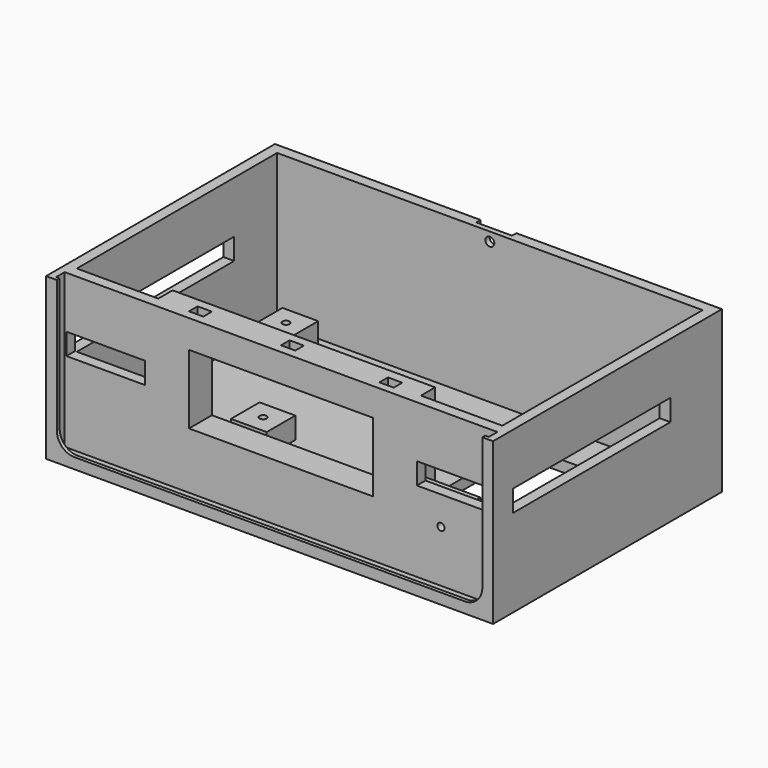
from build123d import *

# Parameters (mm, degrees)
F0_W      = 125
F0_H      = 80
F1_DEPTH  = 45
F3_DEPTH  = 4
F4_W      = 121
F4_H      = 46.7722373752
F5_DEPTH  = 3
F6_W      = 51.45
F6_H      = 19.35
F6_W_2    = 22
F6_H_2    = 6
F7_DEPTH  = 50
F9_DEPTH  = 42
F10_W     = 10
F10_H     = 10
F10_R     = 1
F11_DEPTH = 6
F12_W     = 55
F12_H     = 6
F13_DEPTH = 10
F14_W     = 55
F14_H     = 6
F15_DEPTH = 10
F16_W     = 27.3198820651
F16_H     = 40
F17_DEPTH = 25
F19_W     = 2
F19_H     = 1.5
F20_DEPTH = 5
F21_W     = 27.3198820651
F21_H     = 6
F22_DEPTH = 1.5
F24_R     = 1.5
F25_DEPTH = 10
F26_W     = 4
F26_H     = 3
F27_DEPTH = 5
F28_W     = 10
F28_H     = 10
F29_DEPTH = 1.5
F30_R     = 1.25
F31_DEPTH = 10
F32_W     = 15
F32_H     = 21
F33_DEPTH = 2
F34_R     = 1.4
F34_R_2   = 1.75
F35_DEPTH = 3
F36_R     = 1
F37_DEPTH = 25


# Not quite as in the source:
# - a feature names something its author has since deleted; it is built from what else it names


with BuildPart() as f1:
    # F0 (on Top) → F1 (new body)
    with BuildSketch(Plane.XY):
        Rectangle(F0_W, F0_H)
    extrude(amount=F1_DEPTH)

    # F2 (on face) → F3 (cut)
    with BuildSketch(Plane.XZ.offset(40)):
        with BuildLine():
            Line((-59.5, 47), (-59.5, 7.948817455))
            ThreePointArc((-59.5, 7.948817455), (-58.0505249263, 4.4494750737), (-54.551182545, 3))
            Line((-54.551182545, 3), (0, 3))
            Line((0, 3), (54.551182545, 3))
            ThreePointArc((54.551182545, 3), (58.0505249263, 4.4494750737), (59.5, 7.948817455))
            Line((59.5, 7.948817455), (59.5, 47))
            Line((59.5, 47), (0, 47))
            Line((0, 47), (-59.5, 47))
        make_face()
    extrude(amount=-F3_DEPTH, mode=Mode.SUBTRACT)

    # F4 (on face) → F5 (cut)
    with BuildSketch(Plane.XZ.offset(36)):
        with Locations((0, 25.3861186876)):
            Rectangle(F4_W, F4_H)
    extrude(amount=F5_DEPTH, mode=Mode.SUBTRACT)

    # F6 (on face) → F7 (cut)
    with BuildSketch(Plane.XZ.offset(36)):
        with Locations((0, 27.5)):
            Rectangle(F6_W, F6_H)
        with Locations((-49, 27.5)):
            Rectangle(F6_W_2, F6_H_2)
        with Locations((49, 27.5)):
            Rectangle(F6_W_2, F6_H_2)
    extrude(amount=-F7_DEPTH, mode=Mode.SUBTRACT)

    # F8 (on face) → F9 (cut)
    with BuildSketch(Plane.XY.offset(45)):
        Polygon((-36.725, -28), (0, -28), (0, 37), (-59.5, 37), (-59.5, -33), (-36.725, -33), align=None)
        Polygon((0, 37), (0, -28), (36.725, -28), (36.725, -33), (59.5, -33), (59.5, 37), align=None)
    extrude(amount=-F9_DEPTH, mode=Mode.SUBTRACT)

    # F10 (on face) → F11 (join)
    with BuildSketch(Plane.XY.offset(3)):
        with Locations((-51, 29.5)):
            Rectangle(F10_W, F10_H)
        with Locations((-51, 29.5)):
            Circle(F10_R, mode=Mode.SUBTRACT)
        with Locations((51, 29.5)):
            Rectangle(F10_W, F10_H)
        with Locations((51, 29.5)):
            Circle(F10_R, mode=Mode.SUBTRACT)
        with Locations((51, -22.5)):
            Rectangle(F10_W, F10_H)
        with Locations((51, -22.5)):
            Circle(F10_R, mode=Mode.SUBTRACT)
        with Locations((-27, -8.5)):
            Rectangle(F10_W, F10_H)
        with Locations((-27, -8.5)):
            Circle(F10_R, mode=Mode.SUBTRACT)
    extrude(amount=F11_DEPTH)

    # F12 (on face) → F13 (cut)
    with BuildSketch(Plane(origin=(-62.5, 0, 0), x_dir=(0, -1, 0), z_dir=(-1, 0, 0))):
        with Locations((5.5, 27.5)):
            Rectangle(F12_W, F12_H)
    extrude(amount=-F13_DEPTH, mode=Mode.SUBTRACT)

    # F14 (on face) → F15 (cut)
    with BuildSketch(Plane.YZ.offset(62.5)):
        with Locations((-5.5, 27.5)):
            Rectangle(F14_W, F14_H)
    extrude(amount=-F15_DEPTH, mode=Mode.SUBTRACT)

    # F16 (on face) → F17 (cut)
    with BuildSketch(Plane.XY):
        with Locations((31.5, 5.5)):
            Rectangle(F16_W, F16_H)
    extrude(amount=F17_DEPTH, mode=Mode.SUBTRACT)

    # F19 (on offset) → F20 (cut)
    with BuildSketch(Plane(origin=(0, 25.5, 0), x_dir=(-1, 0, 0), z_dir=(0, 1, 0))):
        with Locations((-22.8400589675, 1.5)):
            Rectangle(F19_W, F19_H)
        with Locations((-40.1599410325, 1.5)):
            Rectangle(F19_W, F19_H)
    extrude(amount=F20_DEPTH, mode=Mode.SUBTRACT)

    # F21 (on face) → F22 (cut)
    with BuildSketch(Plane.XY):
        with Locations((31.5, -17.5)):
            Rectangle(F21_W, F21_H)
    extrude(amount=F22_DEPTH, mode=Mode.SUBTRACT)

    # F24 (on offset) → F25 (cut)
    with BuildSketch(Plane.XY.offset(1.5)):
        with Locations((22.8400589675, -17.5)):
            Circle(F24_R)
        with Locations((40.1599410325, -17.5)):
            Circle(F24_R)
    extrude(amount=F25_DEPTH, mode=Mode.SUBTRACT)

    # F26 (on face) → F27 (cut)
    with BuildSketch(Plane.XY.offset(45)):
        with Locations((0, -32)):
            Rectangle(F26_W, F26_H)
        with Locations((-25.725, -32)):
            Rectangle(F26_W, F26_H)
        with Locations((27.725, -32.2728008032)):
            Rectangle(F26_W, F26_H)
    extrude(amount=-F27_DEPTH, mode=Mode.SUBTRACT)

    # F28 (on face) → F29 (cut)
    with BuildSketch(Plane(origin=(0, 40, 0), x_dir=(-1, 0, 0), z_dir=(0, 1, 0))):
        with Locations((0, 45)):
            Rectangle(F28_W, F28_H)
    extrude(amount=-F29_DEPTH, mode=Mode.SUBTRACT)

    # F30 (on face) → F31 (cut)
    with BuildSketch(Plane(origin=(0, 38.5, 0), x_dir=(-1, 0, 0), z_dir=(0, 1, 0))):
        with Locations((0, 42.5)):
            Circle(F30_R)
    extrude(amount=-F31_DEPTH, mode=Mode.SUBTRACT)

    # F32 (on face) → F33 (join)
    with BuildSketch(Plane(origin=(0, -33, 0), x_dir=(-1, 0, 0), z_dir=(0, 1, 0))):
        with Locations((-44.225, 13.5)):
            Rectangle(F32_W, F32_H)
    extrude(amount=F33_DEPTH)

    # F34 (on face) → F35 (cut)
    with BuildSketch(Plane(origin=(0, -31, 0), x_dir=(-1, 0, 0), z_dir=(0, 1, 0))):
        with Locations((-39.725, 21)):
            Circle(F34_R)
        with Locations((-39.725, 12)):
            Circle(F34_R)
        with Locations((-44.725, 16.5)):
            Circle(F34_R_2)
    extrude(amount=-F35_DEPTH, mode=Mode.SUBTRACT)

    # F36 (on face) → F37 (cut)
    with BuildSketch(Plane(origin=(0, -34, 0), x_dir=(-1, 0, 0), z_dir=(0, 1, 0))):
        with Locations((-44.725, 16.5)):
            Circle(F36_R)
    extrude(amount=-F37_DEPTH, mode=Mode.SUBTRACT)


solid = f1.part
